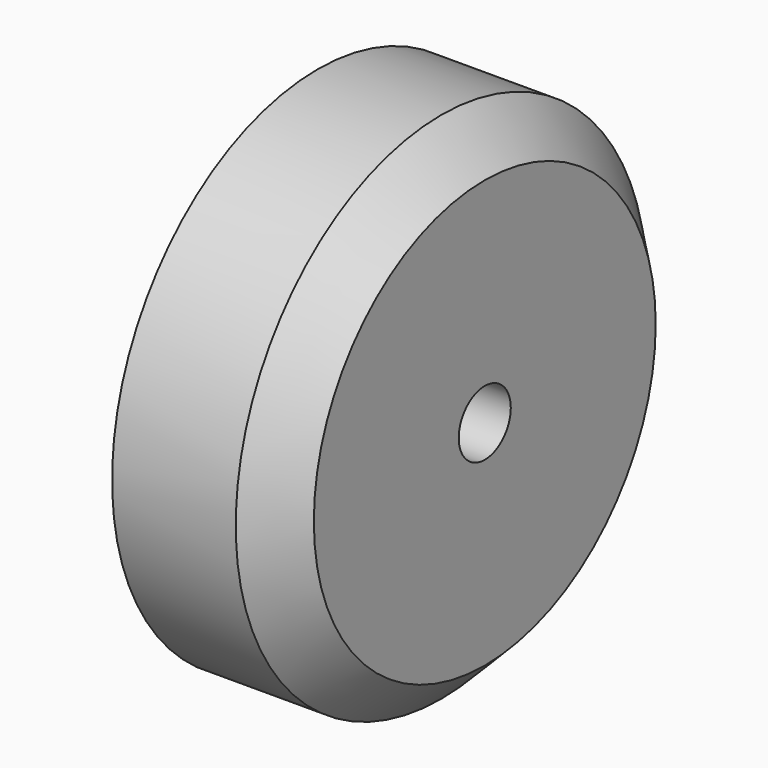
from build123d import *

# Parameters (mm, degrees)
F2_R     = 1.905
F3_DEPTH = 10.542


# Not quite as in the source:
# - a feature names something its author has since deleted; it is built from what else it names


with BuildPart() as f1:
    # F0 (on Front) → F1 (revolve)
    with BuildSketch(Plane.XZ):
        Polygon((8.001, 15.0495), (0.762, 15.0495), (0.762, 13.3985), (7.3171334085, 13.3985), (8.89, 11.8256334085), (8.89, 3.556), (0, 3.556), (0, 0), (10.541, 0), (10.541, 12.5095), align=None)
    revolve(axis=Axis((5.2705, 0, 0), (-1, 0, 0)))

    # F2 (on face) → F3 (cut, through all)
    with BuildSketch(Plane.YZ.offset(10.541)):
        Circle(F2_R)
    extrude(amount=-F3_DEPTH, mode=Mode.SUBTRACT)


solid = f1.part
